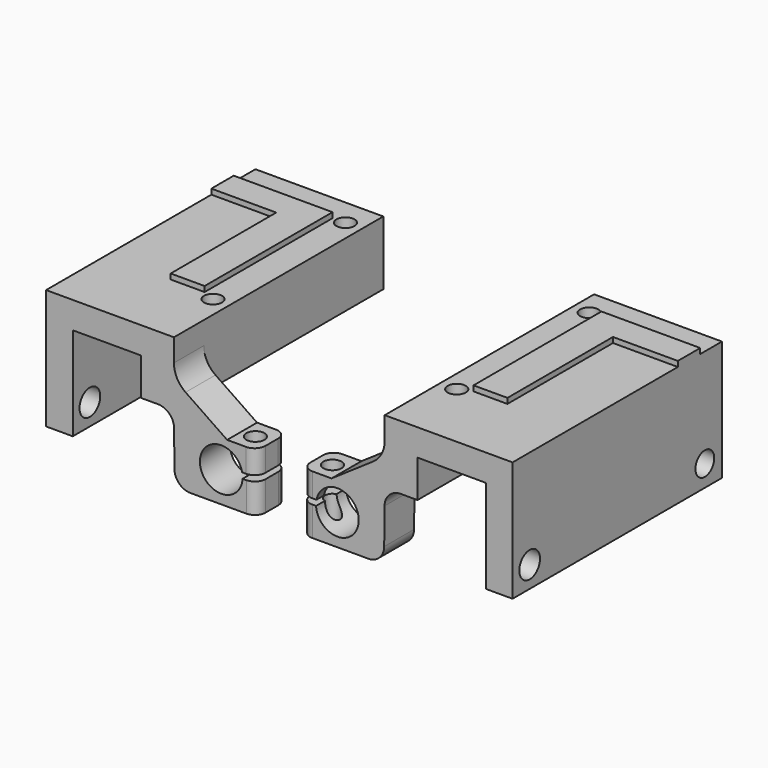
from build123d import *

# Parameters (mm, degrees)
F1_DEPTH      = 7
F2_DEPTH      = 42
F3_R          = 1.7
F3_R_2        = 11
F4_DEPTH      = 12.001
F5_R          = 4
F6_DEPTH      = 10
F7_DEPTH      = 12.001
F8_R          = 1.4
F9_DEPTH      = 10.9920075553
F8_R_2        = 1.7
F10_DEPTH     = 4.4358210087
F11_R         = 5
F12_R         = 3
F13_R         = 3
F14_R         = 2
F15_R         = 2.2
F15_R_2       = 2.4255023423
F16_DEPTH     = 6
F17_TEXT_SIZE = 41.9437823343
F18_DEPTH     = 1


# Not quite as in the source:
# - a feature names something its author has since deleted; it is built from what else it names
# - Text() gives the source's letters only with a copy of the font that has no kerning and outlines rounded to 1/6400 em; it was checked with that copy


with BuildPart() as f1:
    # F0 (on Front) → F1 (new body)
    with BuildSketch(Plane.XZ):
        Polygon((-18.6721007523, 29.8099789735), (-18.6721007523, 7.3259699669), (-13.6721007523, 7.3259699669), (-13.6721007523, 24.8099789735), (-0.8721007523, 24.8099789735), (-0.8721007523, 17.8099789735), (5.2637966118, 17.8099789735), (5.2637966118, 22.9406704692), (5.2637966118, 29.8099789735), align=None)
        Polygon((15.2301751077, 16.1394868046), (5.2637966118, 22.9406704692), (5.2637966118, 17.8099789735), (5.3940201178, 5.1484792493), (20.8186601057, 5.1484792493), (20.8186601057, 10.6682249423), (13.4860510706, 10.6682249423), (13.4860510706, 11.7046658959), (20.7896428882, 11.7046658959), (20.7896428882, 16.1394868046), align=None)
    extrude(amount=F1_DEPTH)

    # F0 (on Front) → F2 (join)
    with BuildSketch(Plane.XZ):
        Polygon((-18.6721007523, 29.8099789735), (-18.6721007523, 7.3259699669), (-13.6721007523, 7.3259699669), (-13.6721007523, 24.8099789735), (-0.8721007523, 24.8099789735), (-0.8721007523, 17.8099789735), (5.2637966118, 17.8099789735), (5.2637966118, 22.9406704692), (5.2637966118, 29.8099789735), align=None)
    extrude(amount=-F2_DEPTH)

    # F3 (on face) → F4 (cut, through all)
    with BuildSketch(Plane(origin=(0, 0, 17.8099789735), x_dir=(1, 0, 0), z_dir=(0, 0, -1))):
        with Locations((2.1850741468, -6)):
            Circle(F3_R)
        with Locations((2.1850741468, -37)):
            Circle(F3_R)
        with Locations((17.6850741468, -21.5)):
            Circle(F3_R_2)
    extrude(amount=-F4_DEPTH, mode=Mode.SUBTRACT)

    # F5 (on face) → F6 (cut)
    with BuildSketch(Plane.XZ.offset(7)):
        with Locations((14.1278992477, 10.8989789735)):
            Circle(F5_R)
    extrude(amount=-F6_DEPTH, mode=Mode.SUBTRACT)

    # F3 (on face) → F7 (cut, through all)
    with BuildSketch(Plane(origin=(0, 0, 17.8099789735), x_dir=(1, 0, 0), z_dir=(0, 0, -1))):
        with Locations((2.1850741468, -6)):
            Circle(F3_R)
        with Locations((2.1850741468, -37)):
            Circle(F3_R)
        with Locations((17.6850741468, -21.5)):
            Circle(F3_R_2)
    extrude(amount=-F7_DEPTH, mode=Mode.SUBTRACT)

    # F8 (on face) → F9 (cut, through all)
    with BuildSketch(Plane.XY.offset(16.1394868046)):
        with Locations((17.7896428882, -3.5767070949)):
            Circle(F8_R)
    extrude(amount=-F9_DEPTH, mode=Mode.SUBTRACT)

    # F8 (on face) → F10 (cut, through all)
    with BuildSketch(Plane.XY.offset(16.1394868046)):
        with Locations((17.7896428882, -3.5767070949)):
            Circle(F8_R_2)
        with Locations((17.7896428882, -3.5767070949)):
            Circle(F8_R, mode=Mode.SUBTRACT)
    extrude(amount=-F10_DEPTH, mode=Mode.SUBTRACT)

    # F11
    f11_edges = [f1.edges().sort_by_distance(p)[0] for p in [
        (5.263797, -3.5, 22.94067),
    ]]
    fillet(f11_edges, radius=F11_R)

    # F12
    f12_edges = [f1.edges().sort_by_distance(p)[0] for p in [
        (5.263797, -3.5, 17.809979),
    ]]
    fillet(f12_edges, radius=F12_R)

    # F13
    f13_edges = [f1.edges().sort_by_distance(p)[0] for p in [
        (5.39402, -3.5, 5.148479),
    ]]
    fillet(f13_edges, radius=F13_R)

    # F14
    f14_edges = [f1.edges().sort_by_distance(p)[0] for p in [
        (20.789643, -7, 13.922076),
        (20.81866, -7, 7.908352),
        (20.789643, 0, 13.922076),
        (20.81866, 0, 7.908352),
    ]]
    fillet(f14_edges, radius=F14_R)

    # F15 (on face) → F16 (cut)
    with BuildSketch(Plane(origin=(-18.6721007523, 0, 0), x_dir=(0, -1, 0), z_dir=(-1, 0, 0))):
        with Locations((-38, 11.3259699669)):
            Circle(F15_R)
        with Locations((3, 11.3259699669)):
            Circle(F15_R_2)
    extrude(amount=-F16_DEPTH, mode=Mode.SUBTRACT)

    # F17 (on face) → F18 (join)
    with BuildSketch(Plane.XY.offset(29.8099789735)):
        with Locations(Location((3.5908724648, 36.9253193088), (0, 0, 180))):
            Text('L', F17_TEXT_SIZE, font='Open Sans', font_style=FontStyle.BOLD, text_align=(TextAlign.LEFT, TextAlign.BOTTOM))
    extrude(amount=F18_DEPTH)


with BuildPart() as f19_1:
    # F19: instance of F1
    add(f1.part.mirror(Plane.YZ))


with BuildPart() as f19_1_1:
    # F20: moved
    add(f19_1.part.moved(Location((50, 0, 0))))


solid = Compound([f1.part, f19_1_1.part])
